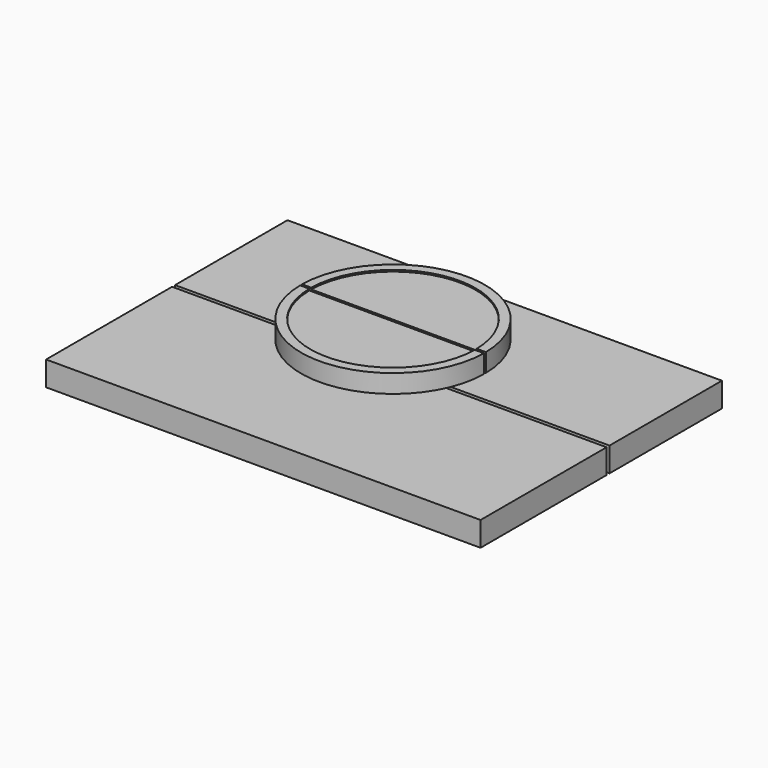
from build123d import *

# Parameters (mm, degrees)
F0_R     = 95.25
F0_R_2   = 85.725
F1_DEPTH = 19.05
F0_R_3   = 28.575
F2_DEPTH = 17.4625
F3_DEPTH = 25.4
F5_DEPTH = 44.451
F6_W     = 450.4083395004
F6_H     = 145.6645973958
F7_DEPTH = 25.4
F6_H_2   = 163.2482669163


# Not quite as in the source:
# - a feature of the source that left no trace in its solid (it failed there, or was rolled back) is left out


with BuildPart() as f1:
    # F0 (on Top) → F1 (new body)
    with BuildSketch(Plane.XY):
        Circle(F0_R)
        Circle(F0_R_2, mode=Mode.SUBTRACT)
    extrude(amount=F1_DEPTH)

    # F0 (on Top) → F2 (join)
    with BuildSketch(Plane.XY):
        Circle(F0_R_2)
        Circle(F0_R_3, mode=Mode.SUBTRACT)
        Circle(F0_R_3)
    extrude(amount=F2_DEPTH)

    # F0 (on Top) → F3 (join)
    with BuildSketch(Plane.XY):
        Circle(F0_R_3)
    extrude(amount=-F3_DEPTH)

    # F4 (on face) → F5 (cut, through all)
    with BuildSketch(Plane(origin=(0, 0, -25.4), x_dir=(1, 0, 0), z_dir=(0, 0, -1))):
        with BuildLine():
            Line((165.4538214207, -1.27), (165.4538214207, 0))
            Line((165.4538214207, 0), (165.4538214207, 1.27))
            Line((165.4538214207, 1.27), (28.5467638271, 1.27))
            ThreePointArc((28.5467638271, 1.27), (28.5679400846, 0.6351569258), (28.575, 0))
            ThreePointArc((28.575, 0), (28.5679400846, -0.6351569258), (28.5467638271, -1.27))
            Line((28.5467638271, -1.27), (165.4538214207, -1.27))
        make_face()
        with BuildLine():
            Line((-28.5467638271, -1.27), (28.5467638271, -1.27))
            ThreePointArc((28.5467638271, -1.27), (28.5679400846, -0.6351569258), (28.575, 0))
            ThreePointArc((28.575, 0), (28.5679400846, 0.6351569258), (28.5467638271, 1.27))
            Line((28.5467638271, 1.27), (-28.5467638271, 1.27))
            ThreePointArc((-28.5467638271, 1.27), (-28.575, 0), (-28.5467638271, -1.27))
        make_face()
        with BuildLine():
            Line((-119.8632493615, -1.27), (-28.5467638271, -1.27))
            ThreePointArc((-28.5467638271, -1.27), (-28.575, 0), (-28.5467638271, 1.27))
            Line((-28.5467638271, 1.27), (-119.8632493615, 1.27))
            Line((-119.8632493615, 1.27), (-119.8632493615, -1.27))
        make_face()
    extrude(amount=-F5_DEPTH, mode=Mode.SUBTRACT)


with BuildPart() as f7:
    # F6 (on face) → F7 (new body)
    with BuildSketch(Plane(origin=(0, 0, -25.4), x_dir=(1, 0, 0), z_dir=(0, 0, -1))):
        with Locations((-2.8137415648, -75.4063900094)):
            Rectangle(F6_W, F6_H)
    extrude(amount=F7_DEPTH)


with BuildPart() as f7b:
    # F6 (on face) → F7, piece 2 (new body)
    with BuildSketch(Plane(origin=(0, 0, -25.4), x_dir=(1, 0, 0), z_dir=(0, 0, -1))):
        with Locations((-2.8137415648, 82.8941334581)):
            Rectangle(F6_W, F6_H_2)
    extrude(amount=F7_DEPTH)


solid = Compound([f1.part, f7.part, f7b.part])
